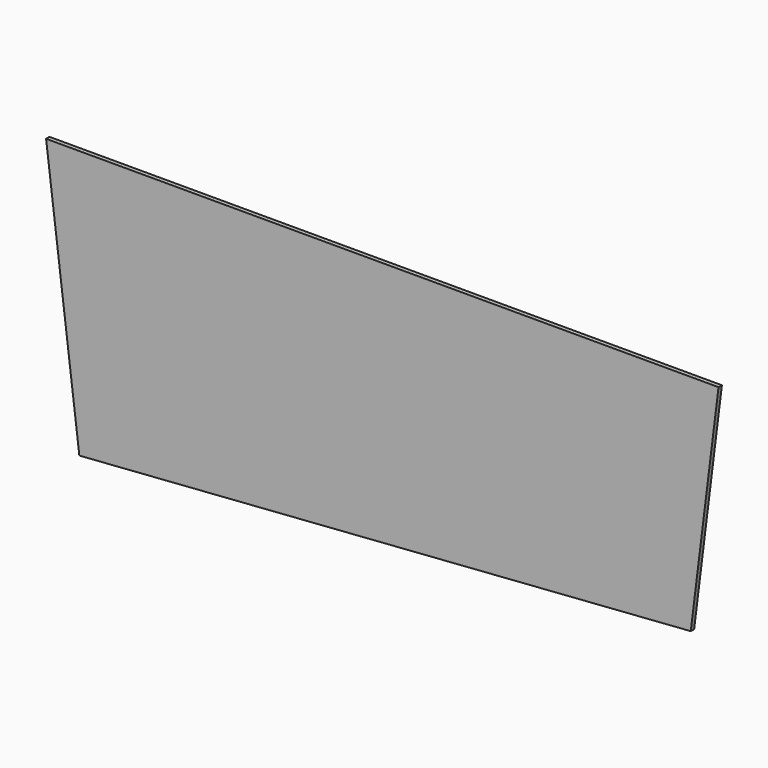
from build123d import *

# Parameters (mm, degrees)
F1_DEPTH = 4.7625


# Not quite as in the source:
# - a length typed as a fraction of an inch, garbled in the dataset ("3 / 203.2 mm" for 3/8 in), is restored


with BuildPart() as f1:
    # F0 (on Front) → F1 (new body)
    with BuildSketch(Plane.XZ):
        Polygon((342.7002896502, -163.4048530862), (380.145872664, 138.4910887061), (-377.0557005115, 138.4910887061), (-345.7904618027, -113.577324326), align=None)
    extrude(amount=F1_DEPTH)


with BuildPart() as f2_1:
    # F2: instance of F1
    add(f1.part.mirror(Plane.YZ))


solid = f2_1.part
